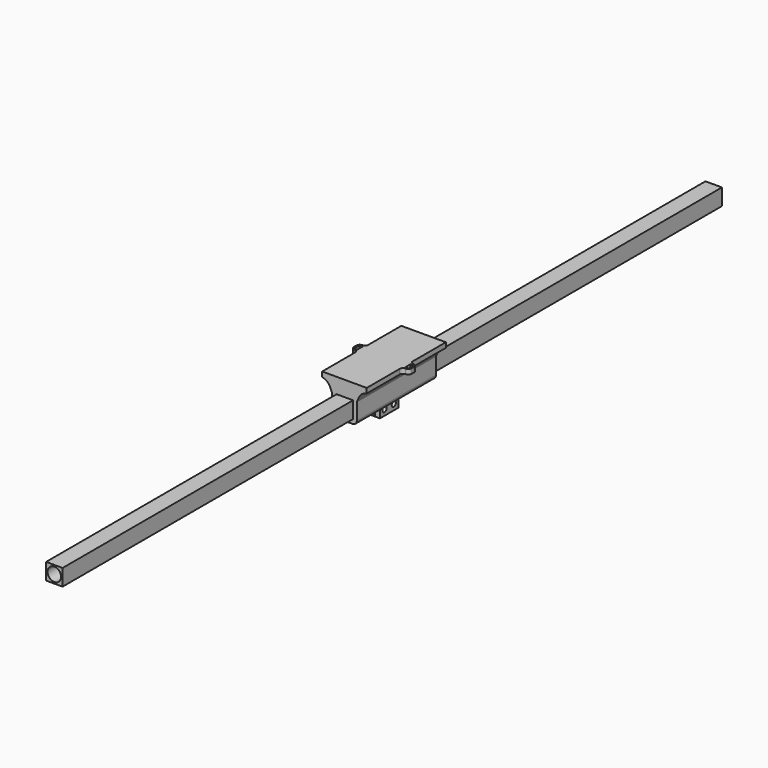
from build123d import *

# Parameters (mm, degrees)
F0_W      = 10
F0_H      = 10
F0_R      = 4.1
F1_DEPTH  = 500
F3_W      = 27
F3_H      = 3
F4_DEPTH  = 30
F3_W_2    = 3
F3_H_2    = 7
F5_DEPTH  = 7
F6_R      = 1.6
F7_DEPTH  = 25
F8_W      = 4
F8_H      = 6
F8_W_2    = 2
F8_H_2    = 4
F9_DEPTH  = 3
F10_R     = 1.99999
F11_W     = 4
F11_H     = 2
F12_DEPTH = 25


# Not quite as in the source:
# - a fillet or chamfer is up to 0.001 mm smaller than in the source, because OpenCascade refuses the exact size


with BuildPart() as f1:
    # F0 (on Front) → F1 (new body)
    with BuildSketch(Plane.XZ):
        Rectangle(F0_W, F0_H)
        Circle(F0_R, mode=Mode.SUBTRACT)
    extrude(amount=F1_DEPTH)


with BuildPart() as f4:
    # F3 (on offset) → F4 (new body, symmetric)
    with BuildSketch(Plane.XZ.offset(250)):
        with BuildLine():
            Line((5, 7.5), (-5, 7.5))
            ThreePointArc((-5, 7.5), (-6.767766953, 6.767766953), (-7.5, 5))
            Line((-7.5, 5), (-7.5, -5))
            ThreePointArc((-7.5, -5), (-6.767766953, -6.767766953), (-5, -7.5))
            Line((-5, -7.5), (-3.15, -7.5))
            Line((-3.15, -7.5), (-0.15, -7.5))
            Line((-0.15, -7.5), (-0.15, -5.2))
            Line((-0.15, -5.2), (-5.2, -5.2))
            Line((-5.2, -5.2), (-5.2, 5.2))
            Line((-5.2, 5.2), (5.2, 5.2))
            Line((5.2, 5.2), (5.2, -5.2))
            Line((5.2, -5.2), (0.15, -5.2))
            Line((0.15, -5.2), (0.15, -7.5))
            Line((0.15, -7.5), (3.15, -7.5))
            Line((3.15, -7.5), (5, -7.5))
            ThreePointArc((5, -7.5), (6.767766953, -6.767766953), (7.5, -5))
            Line((7.5, -5), (7.5, 5))
            ThreePointArc((7.5, 5), (6.767766953, 6.767766953), (5, 7.5))
        make_face()
        with Locations((0, 13)):
            Rectangle(F3_W, F3_H)
        with BuildLine():
            ThreePointArc((-7.5, 5), (-6.767766953, 6.767766953), (-5, 7.5))
            Line((-5, 7.5), (5, 7.5))
            ThreePointArc((5, 7.5), (6.767766953, 6.767766953), (7.5, 5))
            add(Edge.make_bspline(
                [(13.5, 11.5), (8.9917294681, 10.6846382581), (8.3630047739, 6.6367634572), (7.5, 5)],
                knots=[0, 0, 0, 0, 8.8459030065, 8.8459030065, 8.8459030065, 8.8459030065], degree=3))
            Line((13.5, 11.5), (-13.5, 11.5))
            add(Edge.make_bspline(
                [(-13.5, 11.5), (-8.9917294681, 10.6846382581), (-8.3630047739, 6.6367634572), (-7.5, 5)],
                knots=[0, 0, 0, 0, 8.8459030065, 8.8459030065, 8.8459030065, 8.8459030065], degree=3))
        make_face()
    extrude(amount=F4_DEPTH, both=True)

    # F3 (on offset) → F5 (join, symmetric)
    with BuildSketch(Plane.XZ.offset(250)):
        with Locations((-1.65, -11)):
            Rectangle(F3_W_2, F3_H_2)
        with Locations((1.65, -11)):
            Rectangle(F3_W_2, F3_H_2)
    extrude(amount=F5_DEPTH, both=True)

    # F6 (on face) → F7 (cut)
    with BuildSketch(Plane(origin=(-3.15, 0, 0), x_dir=(0, -1, 0), z_dir=(-1, 0, 0))):
        with Locations((246.5, -11)):
            Circle(F6_R)
        with Locations((253.5, -11)):
            Circle(F6_R)
    extrude(amount=-F7_DEPTH, mode=Mode.SUBTRACT)

    # F8 (on face) → F9 (join)
    with BuildSketch(Plane.XY.offset(14.5)):
        with Locations((15.5, -250)):
            Rectangle(F8_W, F8_H)
        with Locations((15.5, -250)):
            Rectangle(F8_W_2, F8_H_2, mode=Mode.SUBTRACT)
        with Locations((-15.5, -250)):
            Rectangle(F8_W, F8_H)
        with Locations((-15.5, -250)):
            Rectangle(F8_W_2, F8_H_2, mode=Mode.SUBTRACT)
    extrude(amount=-F9_DEPTH)

    # F10 (radius 2 in the source; OpenCascade refuses exactly that, so slightly less here)
    f10_edges = [f4.edges().sort_by_distance(p)[0] for p in [
        (-17.5, -247, 13),
        (-13.5, -247, 13),
        (-17.5, -253, 13),
        (-13.5, -253, 13),
        (17.5, -247, 13),
        (13.5, -247, 13),
        (13.5, -253, 13),
        (17.5, -253, 13),
    ]]
    fillet(f10_edges, radius=F10_R)

    # F11 (on face) → F12 (cut)
    with BuildSketch(Plane.YZ.offset(13.5)):
        with Locations((-250, 8.25)):
            Rectangle(F11_W, F11_H)
    extrude(amount=-F12_DEPTH, mode=Mode.SUBTRACT)


solid = Compound([f1.part, f4.part])
